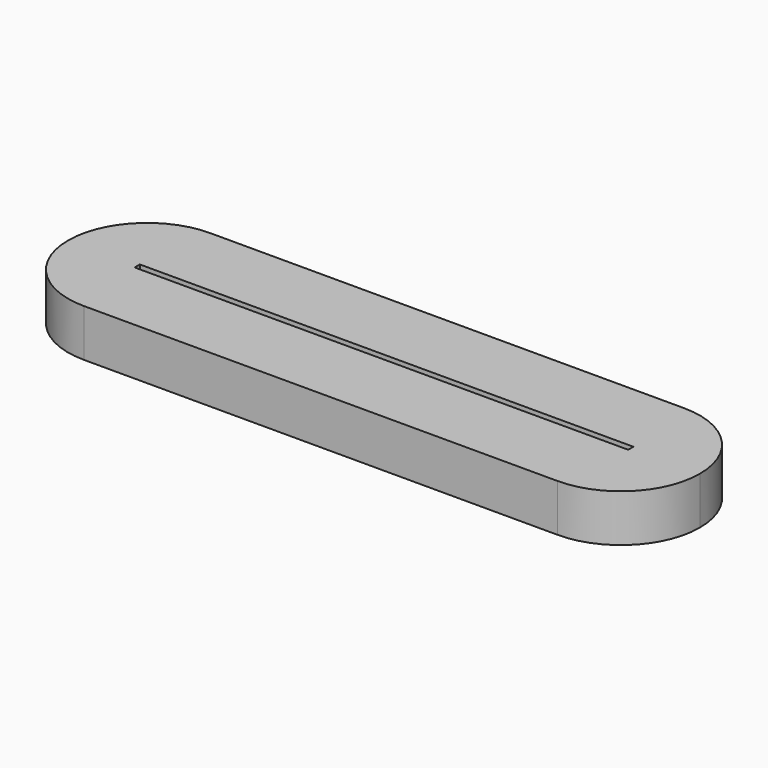
from build123d import *

# Parameters (mm, degrees)
F0_W     = 80
F0_H     = 20
F0_W_2   = 62.5
F0_H_2   = 0.825
F1_DEPTH = 6
F2_R     = 9.99999


# Not quite as in the source:
# - a fillet or chamfer is up to 0.001 mm smaller than in the source, because OpenCascade refuses the exact size


with BuildPart() as f1:
    # F0 (on Top) → F1 (new body)
    with BuildSketch(Plane.XY):
        Rectangle(F0_W, F0_H)
        Rectangle(F0_W_2, F0_H_2, mode=Mode.SUBTRACT)
    extrude(amount=F1_DEPTH)

    # F2 (radius 10 in the source; OpenCascade refuses exactly that, so slightly less here)
    f2_edges = [f1.edges().sort_by_distance(p)[0] for p in [
        (-40, 10, 3),
        (-40, -10, 3),
        (40, 10, 3),
        (40, -10, 3),
    ]]
    fillet(f2_edges, radius=F2_R)


solid = f1.part
